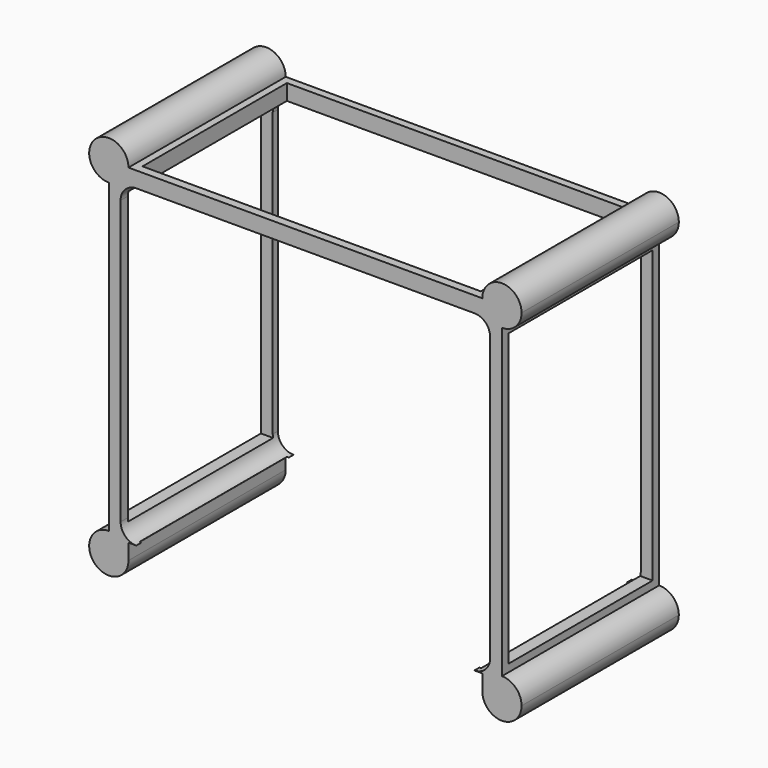
from build123d import *

# Parameters (mm, degrees)
F1_DEPTH       = 63.5
F2_W           = 110.382810235
F2_H           = 59.5524079399
F3_DEPTH       = 25.4
F4_W           = 58.5044906475
F4_H           = 93.9617566764
F5_DEPTH       = 64.77
F6_W           = 109.3032732606
F6_H           = 58.2950827666
F7_DEPTH       = 52.832
F8_W           = 58.2090124954
F8_H           = 93.9617566764
F9_DEPTH       = 43.434
F10_T4_DEPTH   = 63.5
F10_T9_DEPTH   = 76.2
F10_T14_DEPTH  = 76.2
F10_T19_DEPTH  = 76.2
F10_T25_DEPTH  = 76.2
F10_T30_DEPTH  = 76.2
F10_T37_DEPTH  = 76.2
F10_T42_DEPTH  = 88.9
F10_T49_DEPTH  = 76.2
F10_T55_DEPTH  = 76.2
F10_T60_DEPTH  = 76.2
F10_T67_DEPTH  = 76.2
F10_T73_DEPTH  = 76.2
F10_T78_DEPTH  = 76.2
F10_T83_DEPTH  = 76.2
F10_T90_DEPTH  = 88.9
F10_T97_DEPTH  = 76.2
F10_T102_DEPTH = 88.9
F11_W          = 114.3
F11_H          = 5.08
F12_DEPTH      = 127.254


# Not quite as in the source:
# - a fillet or chamfer that OpenCascade refuses, or shapes differently, is made with other operations: its cross-section is extruded or revolved along the edge and cut away or added


with BuildPart() as f1:
    # F0 (on Front) → F1 (new body)
    with BuildSketch(Plane.XZ):
        with BuildLine():
            Line((-62.042625457, -33.4676207812), (-62.042625457, -39.8176207812))
            Line((-62.042625457, -39.8176207812), (-55.692625457, -39.8176207812))
            ThreePointArc((-55.692625457, -39.8176207812), (-56.3630127942, -36.9778144498), (-58.232625457, -34.7376207812))
            ThreePointArc((-58.232625457, -34.7376207812), (-60.0345791428, -33.7934818386), (-62.042625457, -33.4676207812))
        make_face()
        with BuildLine():
            Line((-55.692625457, -39.8176207812), (-62.042625457, -39.8176207812))
            Line((-62.042625457, -39.8176207812), (-62.042625457, -33.4676207812))
            ThreePointArc((-62.042625457, -33.4676207812), (-66.5327535176, -44.3077488417), (-55.692625457, -39.8176207812))
        make_face()
        with BuildLine():
            ThreePointArc((-58.232625457, -34.7376207812), (-56.3630127942, -36.9778144498), (-55.692625457, -39.8176207812))
            Line((-55.692625457, -39.8176207812), (58.607374543, -39.8176207812))
            ThreePointArc((58.607374543, -39.8176207812), (59.2777618801, -36.9778144498), (61.147374543, -34.7376207812))
            Line((61.147374543, -34.7376207812), (-58.232625457, -34.7376207812))
        make_face()
        with BuildLine():
            Line((-62.042625457, 65.5923792188), (-62.042625457, -33.4676207812))
            ThreePointArc((-62.042625457, -33.4676207812), (-60.0345791428, -33.7934818386), (-58.232625457, -34.7376207812))
            Line((-58.232625457, -34.7376207812), (-58.232625457, 66.8623792188))
            ThreePointArc((-58.232625457, 66.8623792188), (-60.0345791428, 65.9182402762), (-62.042625457, 65.5923792188))
        make_face()
        with BuildLine():
            ThreePointArc((61.147374543, -34.7376207812), (59.2777618801, -36.9778144498), (58.607374543, -39.8176207812))
            Line((58.607374543, -39.8176207812), (64.957374543, -39.8176207812))
            Line((64.957374543, -39.8176207812), (64.957374543, -33.4676207812))
            ThreePointArc((64.957374543, -33.4676207812), (62.9493282287, -33.7934818386), (61.147374543, -34.7376207812))
        make_face()
        with BuildLine():
            Line((64.957374543, -39.8176207812), (58.607374543, -39.8176207812))
            ThreePointArc((58.607374543, -39.8176207812), (64.957374543, -46.1676207812), (71.307374543, -39.8176207812))
            ThreePointArc((71.307374543, -39.8176207812), (69.4475026035, -35.3274927207), (64.957374543, -33.4676207812))
            Line((64.957374543, -33.4676207812), (64.957374543, -39.8176207812))
        make_face()
        with BuildLine():
            ThreePointArc((-55.692625457, 71.9423792188), (-66.5327535176, 76.4325072793), (-62.042625457, 65.5923792188))
            Line((-62.042625457, 65.5923792188), (-62.042625457, 71.9423792188))
            Line((-62.042625457, 71.9423792188), (-55.692625457, 71.9423792188))
        make_face()
        with BuildLine():
            Line((-62.042625457, 71.9423792188), (-62.042625457, 65.5923792188))
            ThreePointArc((-62.042625457, 65.5923792188), (-60.0345791428, 65.9182402762), (-58.232625457, 66.8623792188))
            ThreePointArc((-58.232625457, 66.8623792188), (-56.3630127942, 69.1025728874), (-55.692625457, 71.9423792188))
            Line((-55.692625457, 71.9423792188), (-62.042625457, 71.9423792188))
        make_face()
        with BuildLine():
            Line((61.147374543, 66.8623792188), (61.147374543, -34.7376207812))
            ThreePointArc((61.147374543, -34.7376207812), (62.9493282287, -33.7934818386), (64.957374543, -33.4676207812))
            Line((64.957374543, -33.4676207812), (64.957374543, 65.5923792188))
            ThreePointArc((64.957374543, 65.5923792188), (62.9493282287, 65.9182402762), (61.147374543, 66.8623792188))
        make_face()
        with BuildLine():
            ThreePointArc((-55.692625457, 71.9423792188), (-56.3630127942, 69.1025728874), (-58.232625457, 66.8623792188))
            Line((-58.232625457, 66.8623792188), (61.147374543, 66.8623792188))
            ThreePointArc((61.147374543, 66.8623792188), (59.2777618801, 69.1025728874), (58.607374543, 71.9423792188))
            Line((58.607374543, 71.9423792188), (-55.692625457, 71.9423792188))
        make_face()
        with BuildLine():
            ThreePointArc((58.607374543, 71.9423792188), (59.2777618801, 69.1025728874), (61.147374543, 66.8623792188))
            ThreePointArc((61.147374543, 66.8623792188), (62.9493282287, 65.9182402762), (64.957374543, 65.5923792188))
            Line((64.957374543, 65.5923792188), (64.957374543, 71.9423792188))
            Line((64.957374543, 71.9423792188), (58.607374543, 71.9423792188))
        make_face()
        with BuildLine():
            ThreePointArc((71.307374543, 71.9423792188), (64.957374543, 78.2923792188), (58.607374543, 71.9423792188))
            Line((58.607374543, 71.9423792188), (64.957374543, 71.9423792188))
            Line((64.957374543, 71.9423792188), (64.957374543, 65.5923792188))
            ThreePointArc((64.957374543, 65.5923792188), (69.4475026035, 67.4522511583), (71.307374543, 71.9423792188))
        make_face()
    extrude(amount=F1_DEPTH)

    # F2 (on face) → F3 (cut)
    with BuildSketch(Plane(origin=(0, 0, -39.8176207812), x_dir=(1, 0, 0), z_dir=(0, 0, -1))):
        with Locations((1.452460885, 31.7215439281)):
            Rectangle(F2_W, F2_H)
    extrude(amount=-F3_DEPTH, mode=Mode.SUBTRACT)

    # F4 (on face) → F5 (cut)
    with BuildSketch(Plane(origin=(-62.042625457, 0, 0), x_dir=(0, -1, 0), z_dir=(-1, 0, 0))):
        with Locations((31.3205874991, 16.2632633001)):
            Rectangle(F4_W, F4_H)
    extrude(amount=-F5_DEPTH, mode=Mode.SUBTRACT)

    # F6 (on face) → F7 (cut)
    with BuildSketch(Plane.XY.offset(71.9423792188)):
        with Locations((1.3116374612, -31.6250824835)):
            Rectangle(F6_W, F6_H)
    extrude(amount=-F7_DEPTH, mode=Mode.SUBTRACT)

    # F8 (on face) → F9 (cut)
    with BuildSketch(Plane.YZ.offset(64.957374543)):
        with Locations((-31.7638017004, 15.9677881747)):
            Rectangle(F8_W, F8_H)
    extrude(amount=-F9_DEPTH, mode=Mode.SUBTRACT)

    # F10: fillet of radius 5.08 on 4 edges, made by hand


with BuildPart() as f10_tool2:
    # F10_s3 → F10_t4 (new body)
    with BuildSketch(Plane.XZ):
        with BuildLine():
            ThreePointArc((56.067374543, 66.8623792188), (59.6594769914, 65.3744816672), (61.147374543, 61.7823792188))
            Line((61.147374543, 61.7823792188), (61.147374543, 66.8623792188))
            Line((61.147374543, 66.8623792188), (56.067374543, 66.8623792188))
        make_face()
    extrude(amount=F10_T4_DEPTH)

    split(bisect_by=Plane.XY.offset(62.948666513), keep=Keep.TOP)


with BuildPart() as f1_1:
    add(f1.part)

    # F10_t1: union F10_tool2
    add(f10_tool2.part)


with BuildPart() as f10_tool7:
    # F10_s8 → F10_t9 (new body)
    with BuildSketch(Plane.XZ):
        with BuildLine():
            ThreePointArc((56.067374543, 66.8623792188), (59.6594769914, 65.3744816672), (61.147374543, 61.7823792188))
            Line((61.147374543, 61.7823792188), (61.147374543, 66.8623792188))
            Line((61.147374543, 66.8623792188), (56.067374543, 66.8623792188))
        make_face()
    extrude(amount=F10_T9_DEPTH)

    split(bisect_by=Plane.XZ.offset(2.6592954528), keep=Keep.BOTTOM)


with BuildPart() as f1_2:
    add(f1_1.part)

    # F10_t6: union F10_tool7
    add(f10_tool7.part)


with BuildPart() as f10_tool12:
    # F10_s13 → F10_t14 (new body)
    with BuildSketch(Plane.XZ.offset(-12.7)):
        with BuildLine():
            ThreePointArc((56.067374543, 66.8623792188), (59.6594769914, 65.3744816672), (61.147374543, 61.7823792188))
            Line((61.147374543, 61.7823792188), (61.147374543, 66.8623792188))
            Line((61.147374543, 66.8623792188), (56.067374543, 66.8623792188))
        make_face()
    extrude(amount=F10_T14_DEPTH)

    split(bisect_by=Plane.XZ.offset(60.8683079481), keep=Keep.TOP)


with BuildPart() as f1_3:
    add(f1_2.part)

    # F10_t11: union F10_tool12
    add(f10_tool12.part)


with BuildPart() as f10_tool17:
    # F10_s18 → F10_t19 (new body)
    with BuildSketch(Plane.XZ):
        with BuildLine():
            ThreePointArc((-53.152625457, 66.8623792188), (-56.7447279055, 65.3744816672), (-58.232625457, 61.7823792188))
            Line((-58.232625457, 61.7823792188), (-58.232625457, 66.8623792188))
            Line((-58.232625457, 66.8623792188), (-53.152625457, 66.8623792188))
        make_face()
    extrude(amount=F10_T19_DEPTH)

    split(bisect_by=Plane.XZ.offset(2.4775411002), keep=Keep.BOTTOM)

    split(bisect_by=Plane.XY.offset(63.2441416383), keep=Keep.TOP)


with BuildPart() as f1_4:
    add(f1_3.part)

    # F10_t16: union F10_tool17
    add(f10_tool17.part)


with BuildPart() as f10_tool23:
    # F10_s24 → F10_t25 (new body)
    with BuildSketch(Plane.XZ):
        with BuildLine():
            ThreePointArc((-53.152625457, 66.8623792188), (-56.7447279055, 65.3744816672), (-58.232625457, 61.7823792188))
            Line((-58.232625457, 61.7823792188), (-58.232625457, 66.8623792188))
            Line((-58.232625457, 66.8623792188), (-53.152625457, 66.8623792188))
        make_face()
    extrude(amount=F10_T25_DEPTH)

    split(bisect_by=Plane.XZ.offset(2.0683421753), keep=Keep.BOTTOM)


with BuildPart() as f1_5:
    add(f1_4.part)

    # F10_t22: union F10_tool23
    add(f10_tool23.part)


with BuildPart() as f10_tool28:
    # F10_s29 → F10_t30 (new body)
    with BuildSketch(Plane.XZ.offset(-12.7)):
        with BuildLine():
            ThreePointArc((-53.152625457, 66.8623792188), (-56.7447279055, 65.3744816672), (-58.232625457, 61.7823792188))
            Line((-58.232625457, 61.7823792188), (-58.232625457, 66.8623792188))
            Line((-58.232625457, 66.8623792188), (-53.152625457, 66.8623792188))
        make_face()
    extrude(amount=F10_T30_DEPTH)

    split(bisect_by=Plane.YZ.offset(-53.3399991691), keep=Keep.BOTTOM)

    split(bisect_by=Plane.XZ.offset(2.0683421753), keep=Keep.TOP)

    split(bisect_by=Plane.XY.offset(63.2441416383), keep=Keep.TOP)


with BuildPart() as f1_6:
    add(f1_5.part)

    # F10_t27: union F10_tool28
    add(f10_tool28.part)


with BuildPart() as f10_tool35:
    # F10_s36 → F10_t37 (new body)
    with BuildSketch(Plane.XZ.offset(-12.7)):
        with BuildLine():
            ThreePointArc((-53.152625457, 66.8623792188), (-56.7447279055, 65.3744816672), (-58.232625457, 61.7823792188))
            Line((-58.232625457, 61.7823792188), (-58.232625457, 66.8623792188))
            Line((-58.232625457, 66.8623792188), (-53.152625457, 66.8623792188))
        make_face()
    extrude(amount=F10_T37_DEPTH)

    split(bisect_by=Plane.XZ.offset(60.7726238668), keep=Keep.TOP)


with BuildPart() as f1_7:
    add(f1_6.part)

    # F10_t34: union F10_tool35
    add(f10_tool35.part)


with BuildPart() as f10_tool40:
    # F10_s41 → F10_t42 (new body)
    with BuildSketch(Plane.XZ.offset(-12.7)):
        with BuildLine():
            ThreePointArc((-53.152625457, 66.8623792188), (-56.7447279055, 65.3744816672), (-58.232625457, 61.7823792188))
            Line((-58.232625457, 61.7823792188), (-58.232625457, 66.8623792188))
            Line((-58.232625457, 66.8623792188), (-53.152625457, 66.8623792188))
        make_face()
    extrude(amount=F10_T42_DEPTH)

    split(bisect_by=Plane.XZ.offset(60.7726238668), keep=Keep.BOTTOM)

    split(bisect_by=Plane.XZ.offset(60.5728328228), keep=Keep.TOP)

    split(bisect_by=Plane.XY.offset(63.2441416383), keep=Keep.BOTTOM)


with BuildPart() as f1_8:
    add(f1_7.part)

    # F10_t39: union F10_tool40
    add(f10_tool40.part)


with BuildPart() as f10_tool47:
    # F10_s48 → F10_t49 (new body)
    with BuildSketch(Plane.XZ):
        with BuildLine():
            ThreePointArc((61.147374543, -29.6576207812), (59.6594769914, -33.2497232296), (56.067374543, -34.7376207812))
            Line((56.067374543, -34.7376207812), (61.147374543, -34.7376207812))
            Line((61.147374543, -34.7376207812), (61.147374543, -29.6576207812))
        make_face()
    extrude(amount=F10_T49_DEPTH)

    split(bisect_by=Plane.XZ.offset(2.6592954528), keep=Keep.BOTTOM)

    split(bisect_by=Plane.YZ.offset(56.6438660026), keep=Keep.TOP)


with BuildPart() as f1_9:
    add(f1_8.part)

    # F10_t46: union F10_tool47
    add(f10_tool47.part)


with BuildPart() as f10_tool53:
    # F10_s54 → F10_t55 (new body)
    with BuildSketch(Plane.XZ):
        with BuildLine():
            ThreePointArc((61.147374543, -29.6576207812), (59.6594769914, -33.2497232296), (56.067374543, -34.7376207812))
            Line((56.067374543, -34.7376207812), (61.147374543, -34.7376207812))
            Line((61.147374543, -34.7376207812), (61.147374543, -29.6576207812))
        make_face()
    extrude(amount=F10_T55_DEPTH)

    split(bisect_by=Plane.XZ.offset(1.9453399582), keep=Keep.BOTTOM)


with BuildPart() as f1_10:
    add(f1_9.part)

    # F10_t52: union F10_tool53
    add(f10_tool53.part)


with BuildPart() as f10_tool58:
    # F10_s59 → F10_t60 (new body)
    with BuildSketch(Plane.XZ.offset(-12.7)):
        with BuildLine():
            ThreePointArc((61.147374543, -29.6576207812), (59.6594769914, -33.2497232296), (56.067374543, -34.7376207812))
            Line((56.067374543, -34.7376207812), (61.147374543, -34.7376207812))
            Line((61.147374543, -34.7376207812), (61.147374543, -29.6576207812))
        make_face()
    extrude(amount=F10_T60_DEPTH)

    split(bisect_by=Plane.XY.offset(-31.0130901635), keep=Keep.BOTTOM)

    split(bisect_by=Plane.YZ.offset(56.6438660026), keep=Keep.TOP)

    split(bisect_by=Plane.XZ.offset(1.9453399582), keep=Keep.TOP)


with BuildPart() as f1_11:
    add(f1_10.part)

    # F10_t57: union F10_tool58
    add(f10_tool58.part)


with BuildPart() as f10_tool65:
    # F10_s66 → F10_t67 (new body)
    with BuildSketch(Plane.XZ.offset(-12.7)):
        with BuildLine():
            ThreePointArc((61.147374543, -29.6576207812), (59.6594769914, -33.2497232296), (56.067374543, -34.7376207812))
            Line((56.067374543, -34.7376207812), (61.147374543, -34.7376207812))
            Line((61.147374543, -34.7376207812), (61.147374543, -29.6576207812))
        make_face()
    extrude(amount=F10_T67_DEPTH)

    split(bisect_by=Plane.XZ.offset(60.8683079481), keep=Keep.TOP)

    split(bisect_by=Plane.YZ.offset(56.6438660026), keep=Keep.TOP)


with BuildPart() as f1_12:
    add(f1_11.part)

    # F10_t64: union F10_tool65
    add(f10_tool65.part)


with BuildPart() as f10_tool71:
    # F10_s72 → F10_t73 (new body)
    with BuildSketch(Plane.XZ.offset(-12.7)):
        with BuildLine():
            ThreePointArc((61.147374543, -29.6576207812), (59.6594769914, -33.2497232296), (56.067374543, -34.7376207812))
            Line((56.067374543, -34.7376207812), (61.147374543, -34.7376207812))
            Line((61.147374543, -34.7376207812), (61.147374543, -29.6576207812))
        make_face()
    extrude(amount=F10_T73_DEPTH)

    split(bisect_by=Plane.XZ.offset(61.4977478981), keep=Keep.TOP)


with BuildPart() as f1_13:
    add(f1_12.part)

    # F10_t70: union F10_tool71
    add(f10_tool71.part)


with BuildPart() as f10_tool76:
    # F10_s77 → F10_t78 (new body)
    with BuildSketch(Plane.XZ):
        with BuildLine():
            ThreePointArc((-53.152625457, -34.7376207812), (-56.7447279055, -33.2497232296), (-58.232625457, -29.6576207812))
            Line((-58.232625457, -29.6576207812), (-58.232625457, -34.7376207812))
            Line((-58.232625457, -34.7376207812), (-53.152625457, -34.7376207812))
        make_face()
    extrude(amount=F10_T78_DEPTH)

    split(bisect_by=Plane.XZ.offset(1.9453399582), keep=Keep.BOTTOM)


with BuildPart() as f1_14:
    add(f1_13.part)

    # F10_t75: union F10_tool76
    add(f10_tool76.part)


with BuildPart() as f10_tool81:
    # F10_s82 → F10_t83 (new body)
    with BuildSketch(Plane.XZ.offset(-12.7)):
        with BuildLine():
            ThreePointArc((-53.152625457, -34.7376207812), (-56.7447279055, -33.2497232296), (-58.232625457, -29.6576207812))
            Line((-58.232625457, -29.6576207812), (-58.232625457, -34.7376207812))
            Line((-58.232625457, -34.7376207812), (-53.152625457, -34.7376207812))
        make_face()
    extrude(amount=F10_T83_DEPTH)

    split(bisect_by=Plane.XZ.offset(1.9453399582), keep=Keep.TOP)

    split(bisect_by=Plane.YZ.offset(-53.7389442325), keep=Keep.BOTTOM)

    split(bisect_by=Plane.XY.offset(-30.7176150382), keep=Keep.BOTTOM)


with BuildPart() as f1_15:
    add(f1_14.part)

    # F10_t80: union F10_tool81
    add(f10_tool81.part)


with BuildPart() as f10_tool88:
    # F10_s89 → F10_t90 (new body)
    with BuildSketch(Plane.XZ.offset(-12.7)):
        with BuildLine():
            ThreePointArc((-53.152625457, -34.7376207812), (-56.7447279055, -33.2497232296), (-58.232625457, -29.6576207812))
            Line((-58.232625457, -29.6576207812), (-58.232625457, -34.7376207812))
            Line((-58.232625457, -34.7376207812), (-53.152625457, -34.7376207812))
        make_face()
    extrude(amount=F10_T90_DEPTH)

    split(bisect_by=Plane.XZ.offset(1.9453399582), keep=Keep.TOP)

    split(bisect_by=Plane.XY.offset(-30.7176150382), keep=Keep.TOP)

    split(bisect_by=Plane.XZ.offset(2.0683421753), keep=Keep.BOTTOM)


with BuildPart() as f1_16:
    add(f1_15.part)

    # F10_t87: union F10_tool88
    add(f10_tool88.part)


with BuildPart() as f10_tool95:
    # F10_s96 → F10_t97 (new body)
    with BuildSketch(Plane.XZ.offset(-12.7)):
        with BuildLine():
            ThreePointArc((-53.152625457, -34.7376207812), (-56.7447279055, -33.2497232296), (-58.232625457, -29.6576207812))
            Line((-58.232625457, -29.6576207812), (-58.232625457, -34.7376207812))
            Line((-58.232625457, -34.7376207812), (-53.152625457, -34.7376207812))
        make_face()
    extrude(amount=F10_T97_DEPTH)

    split(bisect_by=Plane.XZ.offset(61.4977478981), keep=Keep.TOP)


with BuildPart() as f1_17:
    add(f1_16.part)

    # F10_t94: union F10_tool95
    add(f10_tool95.part)


with BuildPart() as f10_tool100:
    # F10_s101 → F10_t102 (new body)
    with BuildSketch(Plane.XZ.offset(-12.7)):
        with BuildLine():
            ThreePointArc((-53.152625457, -34.7376207812), (-56.7447279055, -33.2497232296), (-58.232625457, -29.6576207812))
            Line((-58.232625457, -29.6576207812), (-58.232625457, -34.7376207812))
            Line((-58.232625457, -34.7376207812), (-53.152625457, -34.7376207812))
        make_face()
    extrude(amount=F10_T102_DEPTH)

    split(bisect_by=Plane.XZ.offset(61.4977478981), keep=Keep.BOTTOM)

    split(bisect_by=Plane.XZ.offset(60.5728328228), keep=Keep.TOP)

    split(bisect_by=Plane.XY.offset(-30.7176150382), keep=Keep.TOP)


with BuildPart() as f1_18:
    add(f1_17.part)

    # F10_t99: union F10_tool100
    add(f10_tool100.part)

    # F11 (on face) → F12 (cut)
    with BuildSketch(Plane.XZ.offset(63.5)):
        with Locations((1.457374543, -37.2776207812)):
            Rectangle(F11_W, F11_H)
    extrude(amount=-F12_DEPTH, mode=Mode.SUBTRACT)


solid = f1_18.part
